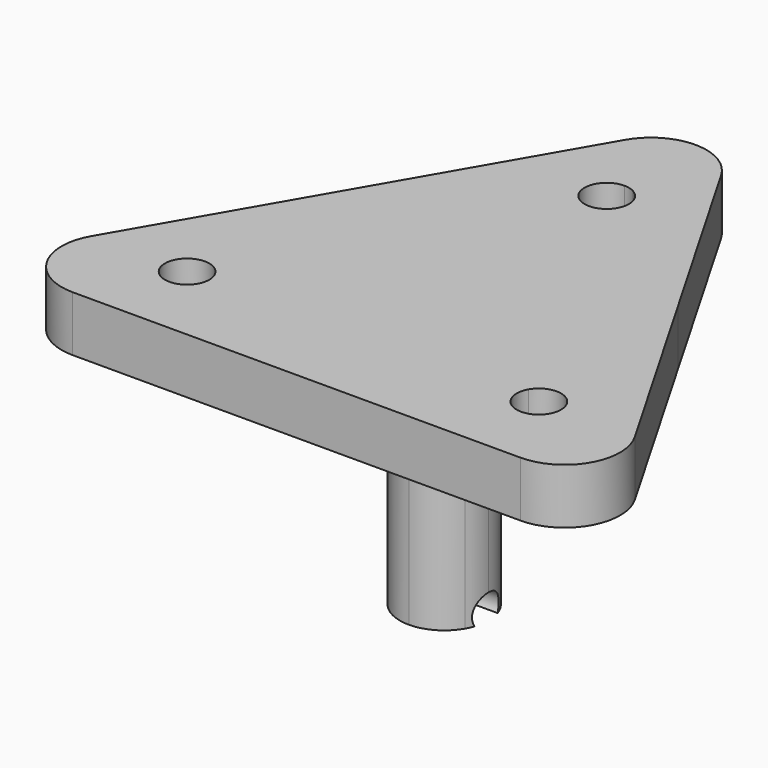
from build123d import *

# Parameters (mm, degrees)
F1_DEPTH = 5
F2_DEPTH = 20
F4_DEPTH = 37.6
F5_SIZE  = 2
F6_R     = 5


# Not quite as in the source:
# - a pattern or mirror of a feature is missing from the dataset's text; its kind, count and spacing are read off the source's solid


with BuildPart() as f1:
    # F0 (on Top) → F1 (new body)
    with BuildSketch(Plane.XY):
        with BuildLine():
            Line((11.2583302492, 6.5), (0, 0))
            Line((0, 0), (28.8675134595, 0))
            Line((28.8675134595, 0), (28.8675134595, 12.6666666667))
            ThreePointArc((28.8675134595, 12.6666666667), (26.8675134595, 13.2025650515), (25.4034118443, 14.6666666667))
            Line((25.4034118443, 14.6666666667), (14.7224318643, 8.5))
            ThreePointArc((14.7224318643, 8.5), (14.9222327093, 8.0176380902), (14.9903810568, 7.5))
            ThreePointArc((14.9903810568, 7.5), (13.508019147, 5.5681483474), (11.2583302492, 6.5))
        make_face()
        with BuildLine():
            Line((14.4337567297, 25), (0, 0))
            Line((0, 0), (11.2583302492, 6.5))
            ThreePointArc((11.2583302492, 6.5), (11.9903810568, 9.2320508076), (14.7224318643, 8.5))
            Line((14.7224318643, 8.5), (25.4034118443, 14.6666666667))
            ThreePointArc((25.4034118443, 14.6666666667), (24.8675134595, 16.6666666667), (25.4034118443, 18.6666666667))
            Line((25.4034118443, 18.6666666667), (14.4337567297, 25))
        make_face()
        with BuildLine():
            Line((28.8675134595, 12.6666666667), (28.8675134595, 0))
            Line((28.8675134595, 0), (57.735026919, 0))
            Line((57.735026919, 0), (46.4766966698, 6.5))
            ThreePointArc((46.4766966698, 6.5), (43.7446458622, 5.7679491924), (43.0125950546, 8.5))
            Line((43.0125950546, 8.5), (32.3316150746, 14.6666666667))
            ThreePointArc((32.3316150746, 14.6666666667), (30.8675134595, 13.2025650515), (28.8675134595, 12.6666666667))
        make_face()
        with BuildLine():
            ThreePointArc((28.8675134595, 20.6666666667), (26.8675134595, 20.1307682818), (25.4034118443, 18.6666666667))
            Line((25.4034118443, 18.6666666667), (28.8675134595, 16.6666666667))
            Line((28.8675134595, 16.6666666667), (28.8675134595, 20.6666666667))
        make_face()
        with BuildLine():
            Line((28.8675134595, 16.6666666667), (25.4034118443, 18.6666666667))
            ThreePointArc((25.4034118443, 18.6666666667), (24.8675134595, 16.6666666667), (25.4034118443, 14.6666666667))
            Line((25.4034118443, 14.6666666667), (28.8675134595, 16.6666666667))
        make_face()
        with BuildLine():
            Line((46.4766966698, 6.5), (57.735026919, 0))
            Line((57.735026919, 0), (43.3012701892, 25))
            Line((43.3012701892, 25), (32.3316150746, 18.6666666667))
            ThreePointArc((32.3316150746, 18.6666666667), (32.7312167646, 17.7019428471), (32.8675134595, 16.6666666667))
            ThreePointArc((32.8675134595, 16.6666666667), (32.7312167646, 15.6313904863), (32.3316150746, 14.6666666667))
            Line((32.3316150746, 14.6666666667), (43.0125950546, 8.5))
            ThreePointArc((43.0125950546, 8.5), (45.2622839524, 9.4318516526), (46.7446458622, 7.5))
            ThreePointArc((46.7446458622, 7.5), (46.6764975148, 6.9823619098), (46.4766966698, 6.5))
        make_face()
        with BuildLine():
            ThreePointArc((25.4034118443, 14.6666666667), (26.8675134595, 13.2025650515), (28.8675134595, 12.6666666667))
            Line((28.8675134595, 12.6666666667), (28.8675134595, 16.6666666667))
            Line((28.8675134595, 16.6666666667), (25.4034118443, 14.6666666667))
        make_face()
        with BuildLine():
            Line((28.8675134595, 16.6666666667), (28.8675134595, 12.6666666667))
            ThreePointArc((28.8675134595, 12.6666666667), (30.8675134595, 13.2025650515), (32.3316150746, 14.6666666667))
            Line((32.3316150746, 14.6666666667), (28.8675134595, 16.6666666667))
        make_face()
        with BuildLine():
            Line((28.8675134595, 20.6666666667), (28.8675134595, 16.6666666667))
            Line((28.8675134595, 16.6666666667), (32.3316150746, 18.6666666667))
            ThreePointArc((32.3316150746, 18.6666666667), (30.8675134595, 20.1307682818), (28.8675134595, 20.6666666667))
        make_face()
        with BuildLine():
            Line((32.3316150746, 18.6666666667), (28.8675134595, 16.6666666667))
            Line((28.8675134595, 16.6666666667), (32.3316150746, 14.6666666667))
            ThreePointArc((32.3316150746, 14.6666666667), (32.7312167646, 15.6313904863), (32.8675134595, 16.6666666667))
            ThreePointArc((32.8675134595, 16.6666666667), (32.7312167646, 17.7019428471), (32.3316150746, 18.6666666667))
        make_face()
    extrude(amount=F1_DEPTH)

    # F1_copies: F1 across plane


with BuildPart() as f1_1:
    add(f1.part)
    add(f1.part.mirror(Plane(origin=(0, 0, 0), x_dir=(0.8660254038, 0.5, 0), z_dir=(-0.5, 0.8660254038, 0))))

    # F0 (on Top) → F2 (join)
    with BuildSketch(Plane.XY):
        with BuildLine():
            Line((32.3316150746, 18.6666666667), (28.8675134595, 16.6666666667))
            Line((28.8675134595, 16.6666666667), (32.3316150746, 14.6666666667))
            ThreePointArc((32.3316150746, 14.6666666667), (32.7312167646, 15.6313904863), (32.8675134595, 16.6666666667))
            ThreePointArc((32.8675134595, 16.6666666667), (32.7312167646, 17.7019428471), (32.3316150746, 18.6666666667))
        make_face()
        with BuildLine():
            Line((28.8675134595, 20.6666666667), (28.8675134595, 16.6666666667))
            Line((28.8675134595, 16.6666666667), (32.3316150746, 18.6666666667))
            ThreePointArc((32.3316150746, 18.6666666667), (30.8675134595, 20.1307682818), (28.8675134595, 20.6666666667))
        make_face()
        with BuildLine():
            ThreePointArc((28.8675134595, 20.6666666667), (26.8675134595, 20.1307682818), (25.4034118443, 18.6666666667))
            Line((25.4034118443, 18.6666666667), (28.8675134595, 16.6666666667))
            Line((28.8675134595, 16.6666666667), (28.8675134595, 20.6666666667))
        make_face()
        with BuildLine():
            Line((28.8675134595, 16.6666666667), (25.4034118443, 18.6666666667))
            ThreePointArc((25.4034118443, 18.6666666667), (24.8675134595, 16.6666666667), (25.4034118443, 14.6666666667))
            Line((25.4034118443, 14.6666666667), (28.8675134595, 16.6666666667))
        make_face()
        with BuildLine():
            ThreePointArc((25.4034118443, 14.6666666667), (26.8675134595, 13.2025650515), (28.8675134595, 12.6666666667))
            Line((28.8675134595, 12.6666666667), (28.8675134595, 16.6666666667))
            Line((28.8675134595, 16.6666666667), (25.4034118443, 14.6666666667))
        make_face()
        with BuildLine():
            Line((28.8675134595, 16.6666666667), (28.8675134595, 12.6666666667))
            ThreePointArc((28.8675134595, 12.6666666667), (30.8675134595, 13.2025650515), (32.3316150746, 14.6666666667))
            Line((32.3316150746, 14.6666666667), (28.8675134595, 16.6666666667))
        make_face()
    extrude(amount=-F2_DEPTH)

    # F3 (on Right) → F4 (cut)
    with BuildSketch(Plane.YZ):
        with BuildLine():
            ThreePointArc((15.165, -19.25), (16.665, -20.75), (18.165, -19.25))
            ThreePointArc((18.165, -19.25), (16.665, -17.75), (15.165, -19.25))
        make_face()
    extrude(amount=F4_DEPTH, mode=Mode.SUBTRACT)

    # F5
    f5_edges = [f1_1.edges().sort_by_distance(p)[0] for p in [
        (10.990381, 7.5, 0),
        (28.867513, 37, 0),
        (46.476697, 6.5, 0),
    ]]
    chamfer(f5_edges, length=F5_SIZE)

    # F6
    f6_edges = [f1_1.edges().sort_by_distance(p)[0] for p in [
        (57.735027, 0, 2.5),
        (0, 0, 2.5),
        (28.867513, 50, 2.5),
    ]]
    fillet(f6_edges, radius=F6_R)


solid = f1_1.part
